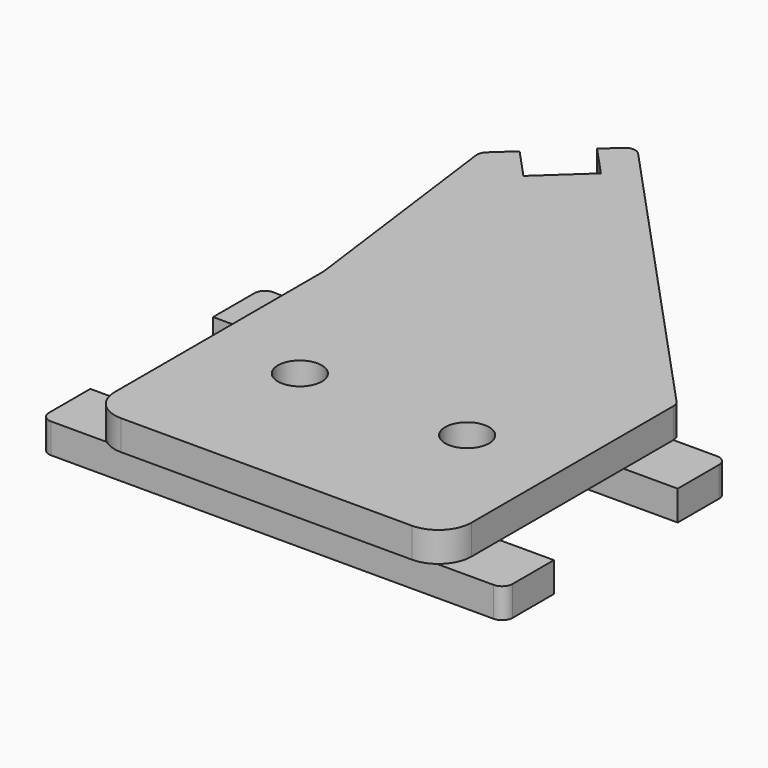
from build123d import *

# Parameters (mm, degrees)
F0_R     = 10.5
F1_DEPTH = 14.2875
F3_DEPTH = 14.2875
F5_DEPTH = 14.2875


# Not quite as in the source:
# - a length typed as a fraction of an inch, garbled in the dataset ("3 / 203.2 mm" for 3/8 in), is restored
# - a feature names something its author has since deleted; it is built from what else it names


with BuildPart() as f1:
    # F0 (on Top) → F1 (new body)
    with BuildSketch(Plane.XY):
        with BuildLine():
            ThreePointArc((-84.5842045546, -55), (-80.1908062724, -65.6066017178), (-69.5842045546, -70))
            Line((-69.5842045546, -70), (69.5842045546, -70))
            ThreePointArc((69.5842045546, -70), (80.7788298305, -65.363034385), (85.4157954454, -54.1684091091))
            Line((85.4157954454, -54.1684091091), (85.4157954454, 66.6648875964))
            ThreePointArc((85.4157954454, 66.6648875964), (85.0717839963, 68.487460123), (84.0870871996, 70.0592383231))
            Line((84.0870871996, 70.0592383231), (-52.4659380977, 217.7534620916))
            ThreePointArc((-52.4659380977, 217.7534620916), (-55.9414029733, 219.3552750765), (-59.5315805785, 218.030403119))
            Line((-59.5315805785, 218.030403119), (-66.8741640868, 211.2417016656))
            Line((-66.8741640868, 211.2417016656), (-53.29676118, 196.556534649))
            Line((-53.29676118, 196.556534649), (-63.9435072671, 186.7129175415))
            Line((-63.9435072671, 186.7129175415), (-74.5902533541, 176.8693004341))
            Line((-74.5902533541, 176.8693004341), (-88.1676562609, 191.5544674507))
            Line((-88.1676562609, 191.5544674507), (-97.2821017235, 183.1275630663))
            ThreePointArc((-97.2821017235, 183.1275630663), (-98.5895263572, 181.1572441104), (-98.845348912, 178.8064844924))
            Line((-98.845348912, 178.8064844924), (-84.6266066394, 70.3235099279))
            ThreePointArc((-84.6266066394, 70.3235099279), (-84.5948163368, 69.9993075241), (-84.5842045546, 69.673723108))
            Line((-84.5842045546, 69.673723108), (-84.5842045546, -55))
        make_face()
        with Locations((-40, 0)):
            Circle(F0_R, mode=Mode.SUBTRACT)
        with Locations((40, 0)):
            Circle(F0_R, mode=Mode.SUBTRACT)
    extrude(amount=F1_DEPTH)

    # F2 (on face) → F3 (join)
    with BuildSketch(Plane(origin=(0, 0, 0), x_dir=(1, 0, 0), z_dir=(0, 0, -1))):
        with BuildLine():
            ThreePointArc((111.2211793661, 61.8855160475), (109.756713272, 65.4210499534), (106.2211793661, 66.8855160475))
            Line((106.2211793661, 66.8855160475), (79.0136510523, 66.8855160475))
            ThreePointArc((79.0136510523, 66.8855160475), (83.7249684911, 61.287261926), (85.4157954454, 54.1684091091))
            Line((85.4157954454, 54.1684091091), (85.4157954454, 37.1908284724))
            Line((85.4157954454, 37.1908284724), (111.2211793661, 37.1908284724))
            Line((111.2211793661, 37.1908284724), (111.2211793661, 61.8855160475))
        make_face()
        with BuildLine():
            ThreePointArc((85.4157954454, 54.1684091091), (83.7249684911, 61.287261926), (79.0136510523, 66.8855160475))
            Line((79.0136510523, 66.8855160475), (-78.7348607215, 66.8855160475))
            ThreePointArc((-78.7348607215, 66.8855160475), (-83.0426562208, 61.623449158), (-84.5842045546, 55))
            Line((-84.5842045546, 55), (-84.5842045546, 37.1908284724))
            Line((-84.5842045546, 37.1908284724), (85.4157954454, 37.1908284724))
            Line((85.4157954454, 37.1908284724), (85.4157954454, 54.1684091091))
        make_face()
        with BuildLine():
            ThreePointArc((-84.5842045546, 55), (-83.0426562208, 61.623449158), (-78.7348607215, 66.8855160475))
            Line((-78.7348607215, 66.8855160475), (-105.4471534491, 66.8855160475))
            ThreePointArc((-105.4471534491, 66.8855160475), (-108.982687355, 65.4210499534), (-110.4471534491, 61.8855160475))
            Line((-110.4471534491, 61.8855160475), (-110.4471534491, 37.1908284724))
            Line((-110.4471534491, 37.1908284724), (-84.5842045546, 37.1908284724))
            Line((-84.5842045546, 37.1908284724), (-84.5842045546, 55))
        make_face()
    extrude(amount=F3_DEPTH)

    # F4 (on face) → F5 (join)
    with BuildSketch(Plane(origin=(0, 0, 0), x_dir=(1, 0, 0), z_dir=(0, 0, -1))):
        with BuildLine():
            Line((111.2211793661, -36.8091715276), (-110.9449085174, -36.8091715276))
            Line((-110.9449085174, -36.8091715276), (-110.9449085174, -61.5038591027))
            ThreePointArc((-110.9449085174, -61.5038591027), (-109.4218951426, -65.0969864325), (-105.7806829141, -66.5011613701))
            Line((-105.7806829141, -66.5011613701), (-102.4463273268, -66.3915849369))
            ThreePointArc((-102.4463273268, -66.3915849369), (-98.8051150983, -67.7957598744), (-97.2821017235, -71.3888872042))
            Line((-97.2821017235, -71.3888872042), (-97.2821017235, -183.1275630663))
            Line((-97.2821017235, -183.1275630663), (-88.1676562609, -191.5544674507))
            Line((-88.1676562609, -191.5544674507), (-74.5902533541, -176.8693004341))
            Line((-74.5902533541, -176.8693004341), (-53.29676118, -196.556534649))
            Line((-53.29676118, -196.556534649), (-66.8741640868, -211.2417016656))
            Line((-66.8741640868, -211.2417016656), (-58.6359989162, -218.8584272777))
            Line((-58.6359989162, -218.8584272777), (58.8349498664, -91.8031638881))
            ThreePointArc((58.8349498664, -91.8031638881), (59.8196466631, -90.2313856879), (60.1636581123, -88.4088131614))
            Line((60.1636581123, -88.4088131614), (60.1636581123, -71.5038591027))
            ThreePointArc((60.1636581123, -71.5038591027), (61.6281242064, -67.9683251968), (65.1636581123, -66.5038591027))
            Line((65.1636581123, -66.5038591027), (106.2211793661, -66.5038591027))
            ThreePointArc((106.2211793661, -66.5038591027), (109.756713272, -65.0393930087), (111.2211793661, -61.5038591027))
            Line((111.2211793661, -61.5038591027), (111.2211793661, -36.8091715276))
        make_face()
    extrude(amount=F5_DEPTH)


solid = f1.part
